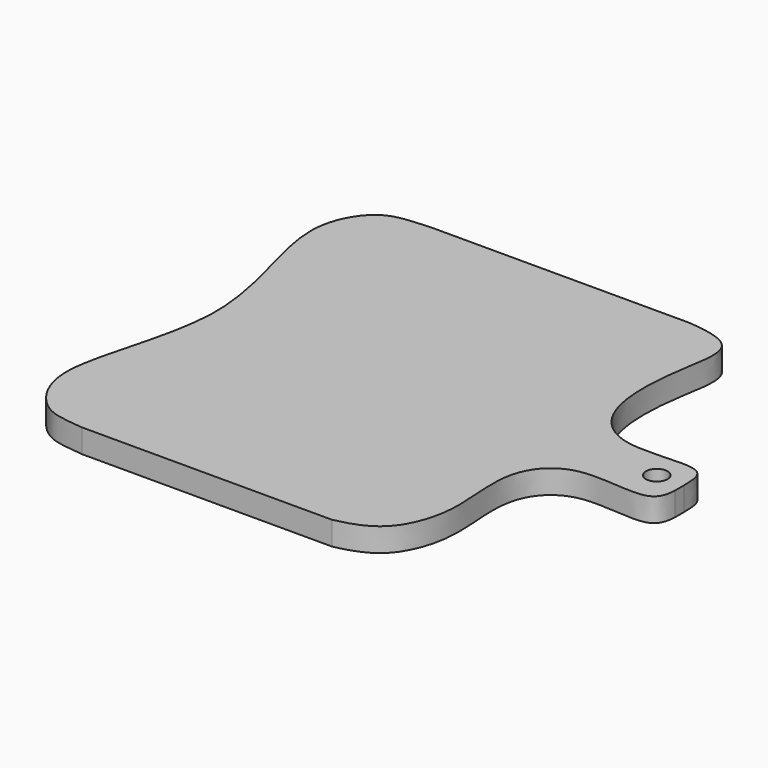
from build123d import *

# Parameters (mm, degrees)
F0_W     = 400
F0_H     = 350
F1_DEPTH = 19
F3_DEPTH = 19.001
F2_R     = 8.68454191
F4_DEPTH = 19.0010001


with BuildPart() as f1:
    # F0 (on Top) → F1 (new body)
    with BuildSketch(Plane.XY):
        Rectangle(F0_W, F0_H)
    extrude(amount=F1_DEPTH)

    # F2 (on face) → F3 (cut, through all)
    with BuildSketch(Plane.XY.offset(19)):
        with BuildLine():
            add(Edge.make_bspline(
                [(-144.3863546874, 175), (-165.2329227667, 173.8789118896), (-183.9453143709, 171.6209800037), (-199.8558619747, 143.6633605964), (-200, 124.4392270745)],
                knots=[0, 0, 0, 0, 0.0401734108, 0.0829469806, 0.0829469806, 0.0829469806, 0.0829469806], degree=3))
            Line((-144.3863546874, 175), (-200, 175))
            Line((-200, 175), (-200, 124.4392270744))
        make_face()
        with BuildLine():
            Line((200, 175), (65.338462454, 175))
            add(Edge.make_bspline(
                [(200, 0), (199.8166252336, 8.7814322248), (199.690280281, 29.6175777687), (133.7661003093, 14.0792968746), (95.3001860897, 49.1740114485), (96.8460076147, 114.6655377081), (109.6455904435, 164.8260868327), (87.5146063822, 172.6839667365), (65.3384624538, 175)],
                knots=[0.6532504807, 0.6532504807, 0.6532504807, 0.6532504807, 0.682714225, 0.7303179586, 0.7734504511, 0.8248457927, 0.8670015807, 0.907356403, 0.907356403, 0.907356403, 0.907356403], degree=3))
            Line((200, 0), (200, 175))
        make_face()
        with BuildLine():
            add(Edge.make_bspline(
                [(-200, 123.3958447292), (-199.7619832828, 91.134165718), (-156.6971429924, 2.4618160265), (-198.7318065847, -87.3217052913), (-200, -118.9837975818)],
                knots=[0.0837173627, 0.0837173627, 0.0837173627, 0.0837173627, 0.1548619144, 0.2226071343, 0.2226071343, 0.2226071343, 0.2226071343], degree=3))
            Line((-200, 123.3958447292), (-200, -118.9837975818))
        make_face()
        with BuildLine():
            add(Edge.make_bspline(
                [(200, -9.1380018675), (200.142398823, -6.1481129118), (200.0631818853, -3.0256477166), (200, 0)],
                knots=[0.6430987301, 0.6430987301, 0.6430987301, 0.6430987301, 0.6532504807, 0.6532504807, 0.6532504807, 0.6532504807], degree=3))
            Line((200, 0), (200, -9.1380018675))
        make_face()
        with BuildLine():
            Line((200, -175), (200, -9.1380018675))
            add(Edge.make_bspline(
                [(56.3706645187, -175), (79.7924420672, -170.2752995484), (98.643784219, -154.1310296062), (110.0260803826, -110.4234542848), (98.5130759268, -54.0890321848), (132.8248140208, -16.3029922353), (195.4041142771, -34.2470777838), (199.6919924438, -15.6051086243), (200, -9.1380018675)],
                knots=[0.3993161169, 0.3993161169, 0.3993161169, 0.3993161169, 0.4430674241, 0.484052229, 0.5315493208, 0.5730877454, 0.6211405717, 0.6430987301, 0.6430987301, 0.6430987301, 0.6430987301], degree=3))
            Line((56.3706645187, -175), (200, -175))
        make_face()
        with BuildLine():
            add(Edge.make_bspline(
                [(-200, -124.838407108), (-199.1662539063, -143.8263247885), (-181.0409866029, -170.2546743415), (-164.3555968809, -173.2601982495), (-144.9777763545, -175)],
                knots=[0.2268886078, 0.2268886078, 0.2268886078, 0.2268886078, 0.2696536718, 0.3085414567, 0.3085414567, 0.3085414567, 0.3085414567], degree=3))
            Line((-200, -124.8384071079), (-200, -175))
            Line((-200, -175), (-144.9777763545, -175))
        make_face()
    extrude(amount=-F3_DEPTH, mode=Mode.SUBTRACT)

    # F2 (on face) → F4 (cut, through all)
    with BuildSketch(Plane.XY.offset(19)):
        with Locations((177.9883056879, 0)):
            Circle(F2_R)
    extrude(amount=-F4_DEPTH, mode=Mode.SUBTRACT)


solid = f1.part
